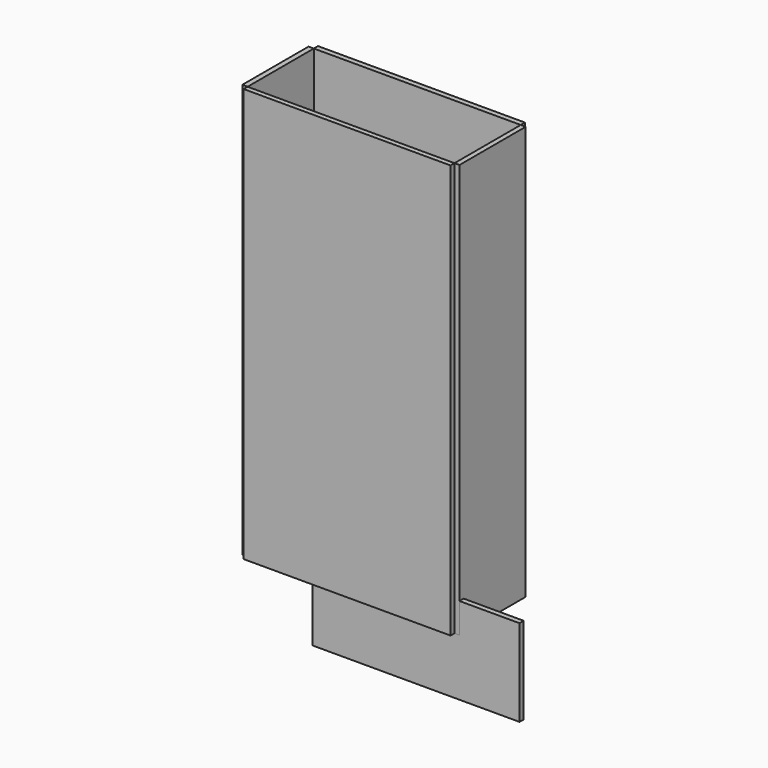
from build123d import *

# Parameters (mm, degrees)
F0_W      = 250
F0_H      = 500
F2_DEPTH  = 6
F7_W      = 100
F7_H      = 500
F8_DEPTH  = 6
F6_W      = 100
F6_H      = 500
F9_DEPTH  = 6.35
F12_W     = 250
F12_H     = 350
F12_R     = 2
F13_DEPTH = 6.35
F15_W     = 250
F15_H     = 105
F16_DEPTH = 6.35
F17_W     = 96
F17_H     = 30
F18_DEPTH = 6


# Not quite as in the source:
# - ends of sketch curves that miss each other by under 0.0002 mm in the source are joined


with BuildPart() as f2:
    # F0 (on Front) → F2 (new body)
    with BuildSketch(Plane.XZ):
        with Locations((-9.2214886099, 172.0402803119)):
            Rectangle(F0_W, F0_H)
    extrude(amount=F2_DEPTH)


with BuildPart() as f8:
    # F7 (on line) → F8 (new body)
    with BuildSketch(Plane(origin=(115.7785113901, 0, 0), x_dir=(0, -1, 0), z_dir=(-1, 0, 0))):
        with Locations((-50, 186.4409143059)):
            Rectangle(F7_W, F7_H)
    extrude(amount=-F8_DEPTH)


with BuildPart() as f9:
    # F6 (on 3pt) → F9 (new body)
    with BuildSketch(Plane.YZ.offset(-134.2214886099)):
        with Locations((62.1549978052, 164.3808417022)):
            Rectangle(F6_W, F6_H)
    extrude(amount=-F9_DEPTH)


with BuildPart() as f9_1:
    # F10: moved
    add(f9.part.moved(Location((0, -12.1549978052, 7.6594386097))))


with BuildPart() as f13:
    # F12 (on face) → F13 (new body)
    with BuildSketch(Plane.XZ.offset(-100)):
        with Locations((-9.2214886099, 247.0402803119)):
            Rectangle(F12_W, F12_H)
        with Locations((-74.2214886099, 139.4918047974)):
            Circle(F12_R, mode=Mode.SUBTRACT)
        Polygon((-5.4219420123, 184.0420639109), (5.1998311024, 186.9017729698), (6.2397954956, 183.0392985561), (-4.382047809, 180.1796009602), align=None, mode=Mode.SUBTRACT)
        Polygon((21.9232730604, 240.9644120841), (32.4612078534, 237.8097440669), (31.3140558471, 233.9777677785), (20.7761210542, 237.1324357958), align=None, mode=Mode.SUBTRACT)
        Polygon((63.6196534227, 202.6301613308), (74.2414265374, 205.4898703897), (75.2813207406, 201.6274074389), (64.659547626, 198.76769838), align=None, mode=Mode.SUBTRACT)
        Polygon((-93.2251735244, 271.2602079822), (-92.0780215182, 275.0921842706), (-81.5400867252, 271.9375162533), (-82.6872387314, 268.105539965), align=None, mode=Mode.SUBTRACT)
    extrude(amount=-F13_DEPTH)


with BuildPart() as f16:
    # F15 (on face) → F16 (new body)
    with BuildSketch(Plane(origin=(0, 0, 0), x_dir=(-1, 0, 0), z_dir=(0, 1, 0))):
        with Locations((-69.3084177162, -94.2262416137)):
            Rectangle(F15_W, F15_H)
    extrude(amount=F16_DEPTH)


with BuildPart() as f18:
    # F17 (on face) → F18 (new body)
    with BuildSketch(Plane(origin=(0, 0, 0), x_dir=(-1, 0, 0), z_dir=(0, 1, 0))):
        with Locations((6.4933296442, 154.4244532514)):
            Rectangle(F17_W, F17_H)
    extrude(amount=F18_DEPTH)


with BuildPart() as f8_1:
    # F19: moved
    add(f8.part.moved(Location((0, 0, -14.400633994))))


solid = Compound([f2.part, f9_1.part, f13.part, f16.part, f18.part, f8_1.part])
